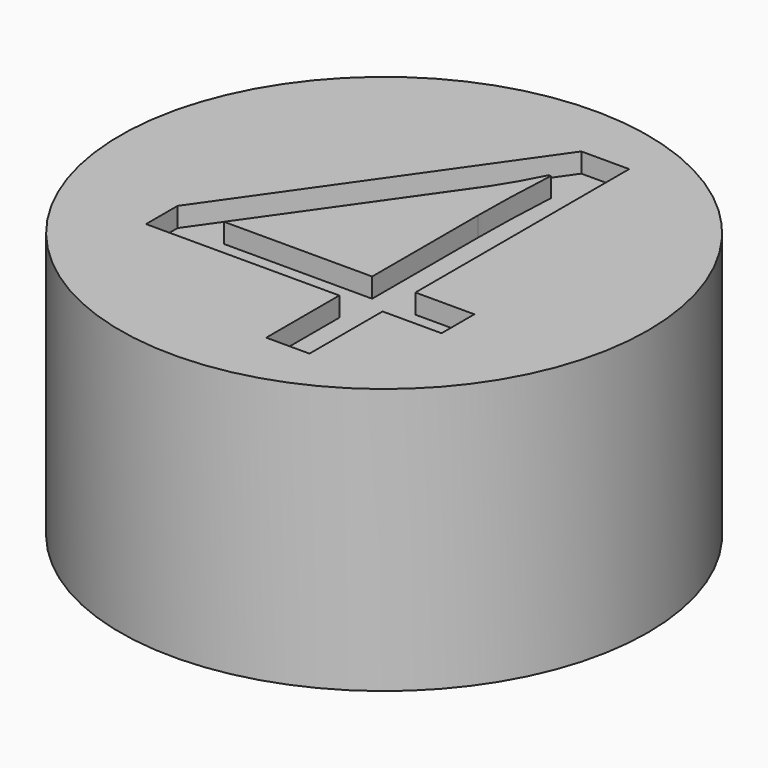
from build123d import *

# Parameters (mm, degrees)
F0_R         = 13.5
F1_DEPTH     = 13.6
F2_TEXT_SIZE = 28.4730157931
F3_DEPTH     = 1


# Not quite as in the source:
# - Text() gives the source's letters only with a copy of the font that has no kerning and outlines rounded to 1/6400 em; it was checked with that copy


with BuildPart() as f1:
    # F0 (on Top) → F1 (new body)
    with BuildSketch(Plane.XY):
        Circle(F0_R)
    extrude(amount=F1_DEPTH)

    # F2 (on face) → F3 (cut)
    with BuildSketch(Plane.XY.offset(13.6)):
        with Locations((-8.4999843129, -10.0124701759)):
            Text('4', F2_TEXT_SIZE, font='Open Sans', text_align=(TextAlign.LEFT, TextAlign.BOTTOM))
    extrude(amount=-F3_DEPTH, mode=Mode.SUBTRACT)


solid = f1.part
